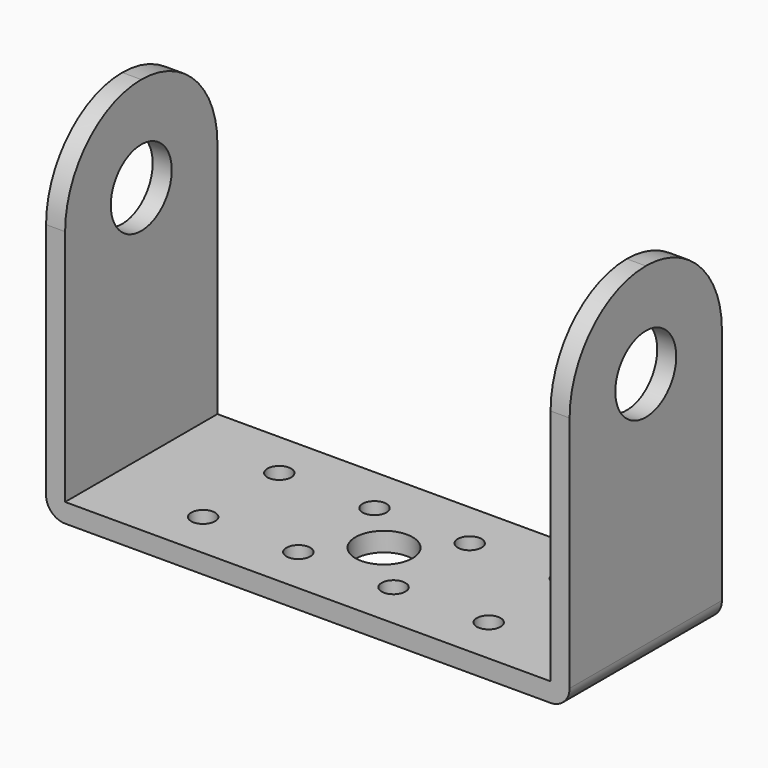
from build123d import *

# Parameters (mm, degrees)
F1_DEPTH = 20
F2_R     = 4
F3_DEPTH = 65.2
F4_R     = 9.99999
F5_R     = 2
F7_D     = 2.5
F8_D     = 6


# Not quite as in the source:
# - a fillet or chamfer is up to 0.001 mm smaller than in the source, because OpenCascade refuses the exact size


with BuildPart() as f1:
    # F0 (on Front) → F1 (new body)
    with BuildSketch(Plane.XZ):
        Polygon((-25.5, 37), (-27.5, 37), (-27.5, 0), (27.5, 0), (27.5, 37), (25.5, 37), (25.5, 2), (-25.5, 2), align=None)
    extrude(amount=F1_DEPTH)

    # F2 (on face) → F3 (cut)
    with BuildSketch(Plane(origin=(-27.5, 0, 0), x_dir=(0, -1, 0), z_dir=(-1, 0, 0))):
        with Locations((10, 27)):
            Circle(F2_R)
    extrude(amount=-F3_DEPTH, mode=Mode.SUBTRACT)

    # F4 (radius 10 in the source; OpenCascade refuses exactly that, so slightly less here)
    f4_edges = [f1.edges().sort_by_distance(p)[0] for p in [
        (-26.5, 0, 37),
        (-26.5, -20, 37),
        (26.5, 0, 37),
        (26.5, -20, 37),
    ]]
    fillet(f4_edges, radius=F4_R)

    # F5
    f5_edges = [f1.edges().sort_by_distance(p)[0] for p in [
        (-27.5, -10, 0),
        (27.5, -10, 0),
    ]]
    fillet(f5_edges, radius=F5_R)

    # F7 (through all)
    with Locations(Plane(origin=(0, 0, 0), x_dir=(1, 0, 0), z_dir=(0, 0, -1))):
        with Locations((-15, 15), (-5, 15), (5, 15), (15, 15), (-15, 5), (-5, 5), (5, 5), (15, 5)):
            Hole(F7_D / 2)

    # F8 (through all)
    with Locations(Plane(origin=(0, 0, 0), x_dir=(1, 0, 0), z_dir=(0, 0, -1))):
        with Locations((0, 10)):
            Hole(F8_D / 2)


solid = f1.part
